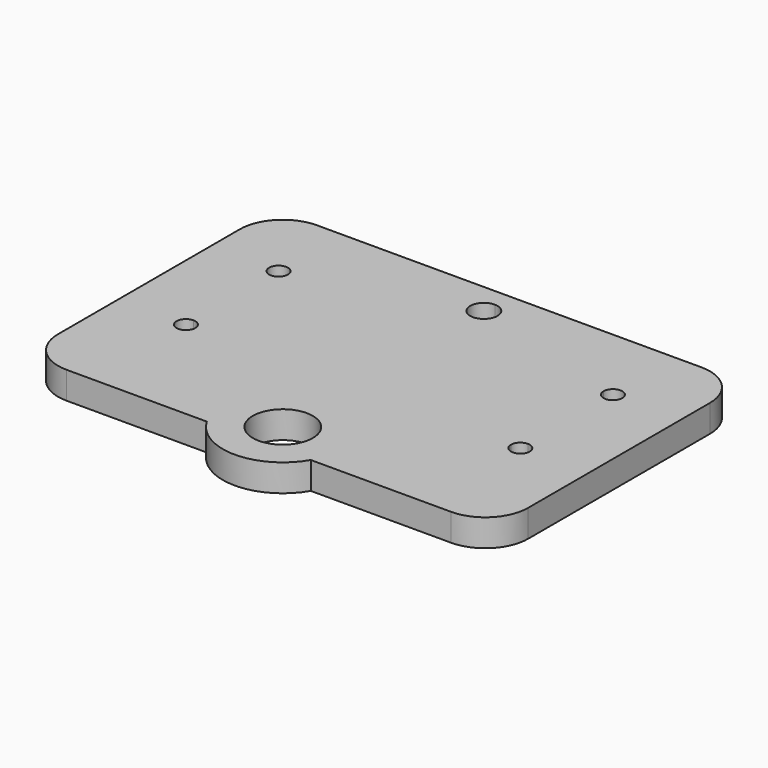
from build123d import *

# Parameters (mm, degrees)
F1_DEPTH = 3.175


# Not quite as in the source:
# - a length typed as a fraction of an inch, garbled in the dataset ("3 / 203.2 mm" for 3/8 in), is restored
# - a feature names something its author has since deleted; it is built from what else it names


with BuildPart() as f1:
    # F0 (on Top) → F1 (new body)
    with BuildSketch(Plane.XY):
        with BuildLine():
            Line((22.4136457592, 16), (0, 16))
            Line((0, 16), (-22.4136457592, 16))
            ThreePointArc((-22.4136457592, 16), (-25.9491796652, 14.5355339059), (-27.4136457592, 11))
            Line((-27.4136457592, 11), (-27.4136457592, -15.5))
            ThreePointArc((-27.4136457592, -15.5), (-25.9491796652, -19.0355339059), (-22.4136457592, -20.5))
            Line((-22.4136457592, -20.5), (-6.0621778265, -20.5))
            ThreePointArc((-6.0621778265, -20.5), (-1.8117333157, -10.238519216), (7, -17))
            ThreePointArc((7, -17), (6.761480784, -18.8117333157), (6.0621778265, -20.5))
            Line((6.0621778265, -20.5), (22.4136457592, -20.5))
            ThreePointArc((22.4136457592, -20.5), (25.9491796652, -19.0355339059), (27.4136457592, -15.5))
            Line((27.4136457592, -15.5), (27.4136457592, 11))
            ThreePointArc((27.4136457592, 11), (25.9491796652, 14.5355339059), (22.4136457592, 16))
        make_face()
        Polygon((22, 9), (22, -9), (-22, -9), (-22, 9), (0, 9), align=None, mode=Mode.SUBTRACT)
        with BuildLine():
            ThreePointArc((1.5875, 12.3080683509), (1.1225320151, 11.1855363358), (0, 10.7205683509))
            ThreePointArc((0, 10.7205683509), (-1.5875, 12.3080683509), (0, 13.8955683509))
            ThreePointArc((0, 13.8955683509), (1.1225320151, 13.4306003661), (1.5875, 12.3080683509))
        make_face(mode=Mode.SUBTRACT)
        Polygon((-22, -9), (22, -9), (22, 9), (0, 9), (-22, 9), align=None)
        with BuildLine():
            Line((-18.4078, 6.75), (0, 6.75))
            Line((0, 6.75), (18.4078, 6.75))
            ThreePointArc((18.4078, 6.75), (19.5, 7.8422), (20.5922, 6.75))
            ThreePointArc((20.5922, 6.75), (20.2723020264, 5.9776979736), (19.5, 5.6578))
            Line((19.5, 5.6578), (19.5, -5.6578))
            ThreePointArc((19.5, -5.6578), (20.2723020264, -5.9776979736), (20.5922, -6.75))
            ThreePointArc((20.5922, -6.75), (19.5, -7.8422), (18.4078, -6.75))
            Line((18.4078, -6.75), (-18.4078, -6.75))
            ThreePointArc((-18.4078, -6.75), (-20.2723020264, -7.5223020264), (-19.5, -5.6578))
            Line((-19.5, -5.6578), (-19.5, 5.6578))
            ThreePointArc((-19.5, 5.6578), (-20.2723020264, 7.5223020264), (-18.4078, 6.75))
        make_face(mode=Mode.SUBTRACT)
        with BuildLine():
            Line((18.4078, 6.75), (0, 6.75))
            Line((0, 6.75), (-18.4078, 6.75))
            ThreePointArc((-18.4078, 6.75), (-18.7276979736, 5.9776979736), (-19.5, 5.6578))
            Line((-19.5, 5.6578), (-19.5, -5.6578))
            ThreePointArc((-19.5, -5.6578), (-18.7276979736, -5.9776979736), (-18.4078, -6.75))
            Line((-18.4078, -6.75), (18.4078, -6.75))
            ThreePointArc((18.4078, -6.75), (18.7276979736, -5.9776979736), (19.5, -5.6578))
            Line((19.5, -5.6578), (19.5, 5.6578))
            ThreePointArc((19.5, 5.6578), (18.7276979736, 5.9776979736), (18.4078, 6.75))
        make_face()
        with BuildLine():
            ThreePointArc((7, -17), (-1.8117333157, -10.238519216), (-6.0621778265, -20.5))
            Line((-6.0621778265, -20.5), (2.55e-08, -20.5))
            Line((2.55e-08, -20.5), (6.0621778265, -20.5))
            ThreePointArc((6.0621778265, -20.5), (6.761480784, -18.8117333157), (7, -17))
        make_face()
        with BuildLine():
            ThreePointArc((3.5, -17), (2.4748737432, -19.4748737251), (2.55e-08, -20.5))
            ThreePointArc((2.55e-08, -20.5), (-2.4748737432, -14.5251262749), (3.5, -17))
        make_face(mode=Mode.SUBTRACT)
        with BuildLine():
            Line((2.55e-08, -20.5), (-6.0621778265, -20.5))
            ThreePointArc((-6.0621778265, -20.5), (0, -24), (6.0621778265, -20.5))
            Line((6.0621778265, -20.5), (2.55e-08, -20.5))
        make_face()
    extrude(amount=F1_DEPTH)


solid = f1.part
